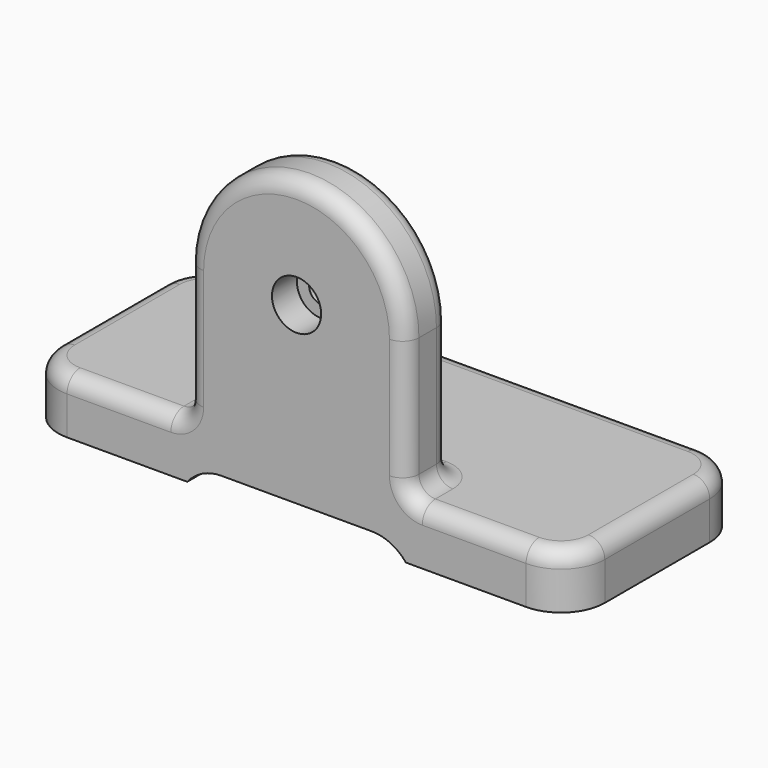
from build123d import *

# Parameters (mm, degrees)
F0_W          = 100
F0_H          = 40
F1_DEPTH      = 10
F3_DEPTH      = 10
F4_W          = 40
F4_H          = 3
F5_DEPTH      = 40.001
F6_R          = 2.25
F7_DEPTH      = 5.7
F8_R          = 2.25
F9_DEPTH      = 40.001
F10_R         = 4.5
F11_DEPTH     = 5.7
F12_T1_DEPTH  = 40
F12_T3_DEPTH  = 40
F12_T5_DEPTH  = 50
F12_T7_DEPTH  = 50
F12_T9_DEPTH  = 50
F12_T11_DEPTH = 50
F13_F1_R      = 3
F13_F2_R      = 3
F13_F3_R      = 3
F14_R         = 14.7416379335
F15_DEPTH     = 10
F16_R         = 5
F17_R         = 4.99999
F19_DEPTH     = 25
F21_DEPTH     = 25
F23_DEPTH     = 25


# Not quite as in the source:
# - a fillet or chamfer that OpenCascade refuses, or shapes differently, is made with other operations: its cross-section is extruded or revolved along the edge and cut away or added
# - a fillet or chamfer is up to 0.001 mm smaller than in the source, because OpenCascade refuses the exact size


with BuildPart() as f1:
    # F0 (on Top) → F1 (new body)
    with BuildSketch(Plane.XY):
        with Locations((-50, 20)):
            Rectangle(F0_W, F0_H)
    extrude(amount=F1_DEPTH)

    # F2 (on Front) → F3 (join)
    with BuildSketch(Plane.XZ):
        with BuildLine():
            Line((-70, 35), (-70, 0))
            Line((-70, 0), (-30, 0))
            Line((-30, 0), (-30, 35))
            ThreePointArc((-30, 35), (-50, 55), (-70, 35))
        make_face()
    extrude(amount=-F3_DEPTH)

    # F4 (on face) → F5 (cut, through all)
    with BuildSketch(Plane.XZ):
        with Locations((-50, 1.5)):
            Rectangle(F4_W, F4_H)
    extrude(amount=-F5_DEPTH, mode=Mode.SUBTRACT)

    # F6 (on face) → F7 (cut)
    with BuildSketch(Plane.XZ):
        with Locations((-50, 35)):
            Circle(F6_R)
    extrude(amount=F7_DEPTH, mode=Mode.SUBTRACT)

    # F8 (on face) → F9 (cut, through all)
    with BuildSketch(Plane.XZ):
        with Locations((-50, 35)):
            Circle(F8_R)
    extrude(amount=-F9_DEPTH, mode=Mode.SUBTRACT)

    # F10 (on face) → F11 (cut)
    with BuildSketch(Plane.XZ):
        with Locations((-50, 35)):
            Circle(F10_R)
    extrude(amount=-F11_DEPTH, mode=Mode.SUBTRACT)

    # F12: fillet of radius 8 on 6 edges, made by hand

    # F12_s2 → F12_t1 (join)
    with BuildSketch(Plane.XZ.offset(-40)):
        with BuildLine():
            ThreePointArc((-70, 0), (-67.2191036167, 2.2111025509), (-63.7550020016, 3))
            Line((-63.7550020016, 3), (-70, 3))
            Line((-70, 3), (-70, 0))
        make_face()
    extrude(amount=F12_T1_DEPTH)

    # F12_s4 → F12_t3 (join)
    with BuildSketch(Plane.XZ.offset(-40)):
        with BuildLine():
            ThreePointArc((-36.2449979984, 3), (-32.7808963833, 2.2111025509), (-30, 0))
            Line((-30, 0), (-30, 3))
            Line((-30, 3), (-36.2449979984, 3))
        make_face()
    extrude(amount=F12_T3_DEPTH)

    # F12_s6 → F12_t5 (cut)
    with BuildSketch(Plane.XY.offset(-20)):
        with BuildLine():
            ThreePointArc((-92, 0), (-97.6568542495, 2.3431457505), (-100, 8))
            Line((-100, 8), (-100, 0))
            Line((-100, 0), (-92, 0))
        make_face()
    extrude(amount=F12_T5_DEPTH, mode=Mode.SUBTRACT)

    # F12_s8 → F12_t7 (cut)
    with BuildSketch(Plane.XY.offset(-20)):
        with BuildLine():
            ThreePointArc((-8, 0), (-2.3431457505, 2.3431457505), (0, 8))
            Line((0, 8), (0, 0))
            Line((0, 0), (-8, 0))
        make_face()
    extrude(amount=F12_T7_DEPTH, mode=Mode.SUBTRACT)

    # F12_s10 → F12_t9 (cut)
    with BuildSketch(Plane.XY.offset(-20)):
        with BuildLine():
            ThreePointArc((-100, 32), (-97.6568542495, 37.6568542495), (-92, 40))
            Line((-92, 40), (-100, 40))
            Line((-100, 40), (-100, 32))
        make_face()
    extrude(amount=F12_T9_DEPTH, mode=Mode.SUBTRACT)

    # F12_s12 → F12_t11 (cut)
    with BuildSketch(Plane.XY.offset(-20)):
        with BuildLine():
            ThreePointArc((-8, 40), (-2.3431457505, 37.6568542495), (0, 32))
            Line((0, 32), (0, 40))
            Line((0, 40), (-8, 40))
        make_face()
    extrude(amount=F12_T11_DEPTH, mode=Mode.SUBTRACT)

    # F13: fillet of radius 3 on 19 edges, made by hand

    # F13_f1
    f13_f1_edges = [f1.edges().sort_by_distance(p)[0] for p in [
        (-50, 10, 55),
        (-30, 10, 22.5),
        (-70, 10, 22.5),
    ]]
    fillet(f13_f1_edges, radius=F13_F1_R)

    # F13_f2
    f13_f2_edges = [f1.edges().sort_by_distance(p)[0] for p in [
        (-30, 3.5, 10),
        (-50, 10, 10),
        (-69.1213203436, 9.1213203436, 10),
        (-30.8786796564, 9.1213203436, 10),
    ]]
    fillet(f13_f2_edges, radius=F13_F2_R)

    # F13_f3
    f13_f3_edges = [f1.edges().sort_by_distance(p)[0] for p in [
        (-50, 0, 55),
        (-17.5, 0, 10),
        (-30, 0, 24),
        (-70, 0, 24),
        (-82.5, 0, 10),
        (-2.3431457505, 2.3431457505, 10),
        (-97.6568542495, 2.3431457505, 10),
        (-100, 20, 10),
        (-97.6568542495, 37.6568542495, 10),
        (-50, 40, 10),
        (-2.3431457505, 37.6568542495, 10),
        (0, 20, 10),
        (-70.8786796564, 0, 10.8786796564),
        (-29.1213203436, 0, 10.8786796564),
    ]]
    fillet(f13_f3_edges, radius=F13_F3_R)


with BuildPart() as f15:
    # F14 (on Front) → F15 (new body)
    with BuildSketch(Plane.XZ):
        with Locations((13.6165842414, 30.4193142802)):
            Circle(F14_R)
    extrude(amount=F15_DEPTH)

    # F16
    f16_edges = [f15.edges().sort_by_distance(p)[0] for p in [
        (-1.125054, 0, 30.419314),
    ]]
    fillet(f16_edges, radius=F16_R)

    # F17 (radius 5 in the source; OpenCascade refuses exactly that, so slightly less here)
    f17_edges = [f15.edges().sort_by_distance(p)[0] for p in [
        (-1.125054, -10, 30.419314),
    ]]
    fillet(f17_edges, radius=F17_R)

    # F18 (on face) → F19 (cut)
    with BuildSketch(Plane(origin=(0, 0, 0), x_dir=(-1, 0, 0), z_dir=(0, 1, 0))):
        with BuildLine():
            add(Edge.make_bspline(
                [(-19.4401461631, 32.8323282301), (-19.9968709509, 33.2770508944), (-19.4875302189, 34.8962578968), (-18.1048562016, 35.5958145992), (-15.3783069075, 36.2560620537), (-15.8567536171, 32.5328810398), (-15.7555112506, 32.3441027388), (-18.6503721636, 32.2014412912), (-19.4401461631, 32.8323282301)],
                knots=[0, 0, 0, 0, 0.1670809127, 0.3308667094, 0.503547456, 0.7173756393, 0.7629777521, 1, 1, 1, 1], degree=3))
        make_face()
    extrude(amount=-F19_DEPTH, mode=Mode.SUBTRACT)

    # F20 (on face) → F21 (cut)
    with BuildSketch(Plane(origin=(0, 0, 0), x_dir=(-1, 0, 0), z_dir=(0, 1, 0))):
        with BuildLine():
            add(Edge.make_bspline(
                [(-19.2039739341, 28.8294907659), (-19.9554901329, 27.9470783872), (-15.441516591, 25.1571436159), (-11.3543379993, 24.1565995472), (-3.9958502764, 30.6267965352), (-18.0118143302, 30.2292961108), (-19.2039739341, 28.8294907659)],
                knots=[0, 0, 0, 0, 0.2137062215, 0.4441739077, 0.6609894441, 1, 1, 1, 1], degree=3))
        make_face()
    extrude(amount=-F21_DEPTH, mode=Mode.SUBTRACT)

    # F22 (on face) → F23 (cut)
    with BuildSketch(Plane(origin=(0, 0, 0), x_dir=(-1, 0, 0), z_dir=(0, 1, 0))):
        with BuildLine():
            add(Edge.make_bspline(
                [(-11.5732420236, 32.4865654111), (-10.5787623693, 32.5525718403), (-7.6674853918, 31.6142853476), (-7.6892600681, 35.1157007314), (-12.2106904501, 36.948425314), (-13.1456057302, 31.8178145815), (-12.1437595998, 32.4486985449), (-11.5732420236, 32.4865654111)],
                knots=[0, 0, 0, 0, 0.2273765403, 0.4100675561, 0.6434669892, 0.8695576002, 1, 1, 1, 1], degree=3))
        make_face()
    extrude(amount=-F23_DEPTH, mode=Mode.SUBTRACT)


solid = f1.part
